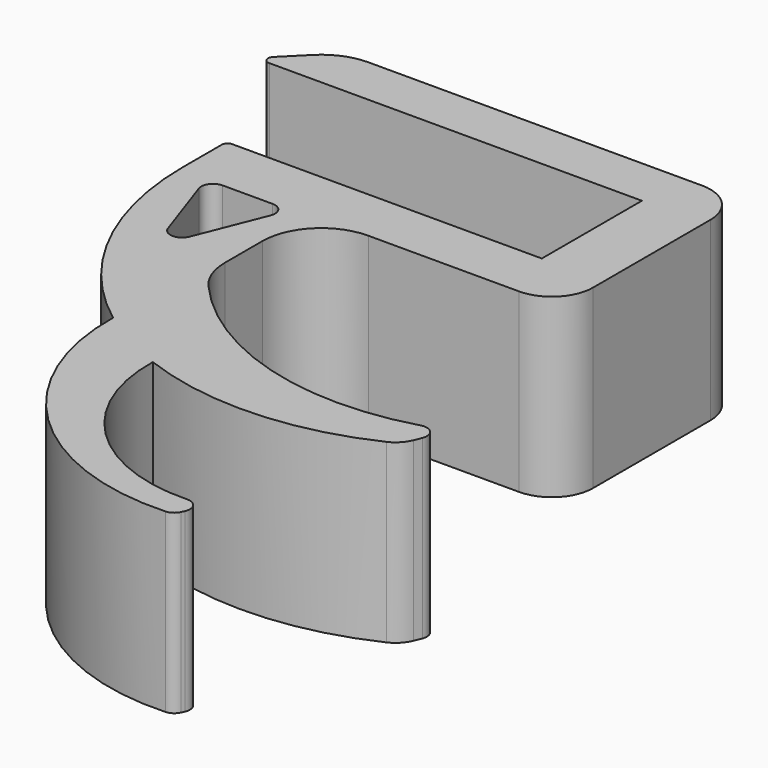
from build123d import *

# Parameters (mm, degrees)
F0_W        = 10.5280357461
F0_H        = 21.2543252856
F1_DEPTH    = 30
F2_R        = 5
F3_R        = 2
F4_R        = 2
F5_R        = 2
F6_R        = 7
F7_T1_DEPTH = 81.4336597593
F8_R        = 10
F9_R        = 1
F10_R       = 10
F11_R       = 10
F13_DEPTH   = 30
F14_R       = 2


# Not quite as in the source:
# - a fillet or chamfer that OpenCascade refuses, or shapes differently, is made with other operations: its cross-section is extruded or revolved along the edge and cut away or added


with BuildPart() as f1:
    # F0 (on Top) → F1 (new body)
    with BuildSketch(Plane.XY):
        Polygon((23.4277165425, 17.0276444405), (-54.4175144403, 17.0276444405), (-54.4175144403, 8.6288927123), (12.8996807964, 8.6288927123), (23.4277165425, 8.6288927123), align=None)
        with Locations((18.1636986695, -1.9982699305)):
            Rectangle(F0_W, F0_H)
        Polygon((23.4277165425, -21.8901360014), (23.4277165425, -12.6254325733), (12.8996807964, -12.6254325733), (-40.6902853517, -12.6254325733), (-40.6902853517, -21.8901360014), (-27.7488247443, -21.8901360014), (-19.1767220313, -21.8901360014), align=None)
        with BuildLine():
            Line((-19.1767220313, -43.3673763092), (-19.1767220313, -21.8901360014))
            Line((-19.1767220313, -21.8901360014), (-27.7488247443, -21.8901360014))
            ThreePointArc((-27.7488247443, -21.8901360014), (-24.844212154, -33.1801228498), (-19.1767220313, -43.3673763092))
        make_face()
        with BuildLine():
            Line((-27.7488247443, -21.8901360014), (-40.6902853517, -21.8901360014))
            ThreePointArc((-40.6902853517, -21.8901360014), (-35.4626283769, -44.0139601174), (-20.8854291365, -61.4580781309))
            ThreePointArc((-20.8854291365, -61.4580781309), (-15.0806794225, -65.2011539101), (-8.8108392586, -68.098538912))
            ThreePointArc((-8.8108392586, -68.098538912), (11.6035028188, -71.235670703), (31.5175838768, -65.7569542527))
            Line((31.5175838768, -65.7569542527), (34.4113459094, -58.7176481952))
            ThreePointArc((34.4113459094, -58.7176481952), (5.0047282318, -60.1630877212), (-19.1767220313, -43.3673763092))
            ThreePointArc((-19.1767220313, -43.3673763092), (-24.844212154, -33.1801228498), (-27.7488247443, -21.8901360014))
        make_face()
        with BuildLine():
            ThreePointArc((-8.8108392586, -68.098538912), (-15.0806794225, -65.2011539101), (-20.8854291365, -61.4580781309))
            ThreePointArc((-20.8854291365, -61.4580781309), (-8.8309401238, -90.1622048174), (20.5386656224, -100.4900241667))
            Line((20.5386656224, -100.4900241667), (22.6970568086, -95.7385333169))
            ThreePointArc((22.6970568086, -95.7385333169), (0.4530333538, -89.3168234963), (-8.8108392586, -68.098538912))
        make_face()
    extrude(amount=F1_DEPTH)

    # F2
    f2_edges = [f1.edges().sort_by_distance(p)[0] for p in [
        (31.517584, -65.756954, 15),
    ]]
    fillet(f2_edges, radius=F2_R)

    # F3
    f3_edges = [f1.edges().sort_by_distance(p)[0] for p in [
        (34.411346, -58.717648, 15),
    ]]
    fillet(f3_edges, radius=F3_R)

    # F4
    f4_edges = [f1.edges().sort_by_distance(p)[0] for p in [
        (22.697057, -95.738533, 15),
    ]]
    fillet(f4_edges, radius=F4_R)

    # F5
    f5_edges = [f1.edges().sort_by_distance(p)[0] for p in [
        (20.538666, -100.490024, 15),
    ]]
    fillet(f5_edges, radius=F5_R)

    # F6
    f6_edges = [f1.edges().sort_by_distance(p)[0] for p in [
        (23.427717, -21.890136, 15),
        (23.427717, 17.027644, 15),
    ]]
    fillet(f6_edges, radius=F6_R)

    # F7: chamfer of 10 on 1 edges, made by hand

    # F7_s2 → F7_t1 (cut)
    with BuildSketch(Plane.XY.offset(-25.7168298797)):
        Polygon((-44.4175144403, 17.0276444405), (-54.4175144403, 7.0276444405), (-54.4175144403, 17.0276444405), align=None)
    extrude(amount=F7_T1_DEPTH, mode=Mode.SUBTRACT)

    # F8
    f8_edges = [f1.edges().sort_by_distance(p)[0] for p in [
        (-44.417514, 17.027644, 15),
    ]]
    fillet(f8_edges, radius=F8_R)

    # F9
    f9_edges = [f1.edges().sort_by_distance(p)[0] for p in [
        (-52.816266, 8.628893, 15),
        (-40.690285, -12.625433, 15),
    ]]
    fillet(f9_edges, radius=F9_R)

    # F10
    f10_edges = [f1.edges().sort_by_distance(p)[0] for p in [
        (-19.176722, -21.890136, 15),
    ]]
    fillet(f10_edges, radius=F10_R)

    # F11
    f11_edges = [f1.edges().sort_by_distance(p)[0] for p in [
        (-19.176722, -43.367376, 15),
    ]]
    fillet(f11_edges, radius=F11_R)

    # F12 (on face) → F13 (cut)
    with BuildSketch(Plane.XY.offset(30)):
        Polygon((-21.8362864107, -22.6786807179), (-36.1205674708, -22.6786807179), (-29.5046903193, -41.924867779), align=None)
    extrude(amount=-F13_DEPTH, mode=Mode.SUBTRACT)

    # F14
    f14_edges = [f1.edges().sort_by_distance(p)[0] for p in [
        (-21.836286, -22.678681, 15),
        (-36.120567, -22.678681, 15),
        (-29.50469, -41.924868, 15),
    ]]
    fillet(f14_edges, radius=F14_R)


solid = f1.part
